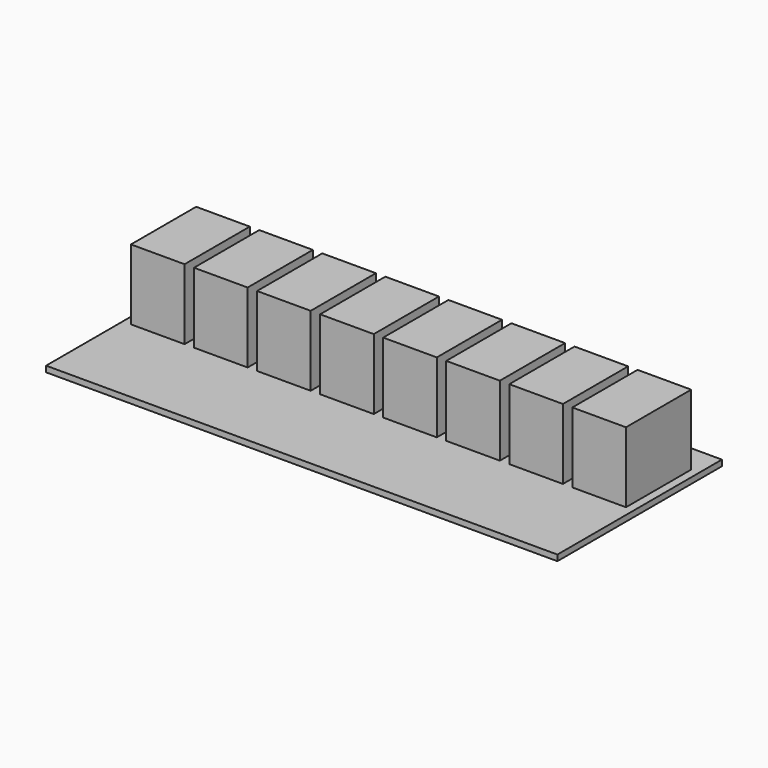
from build123d import *

# Parameters (mm, degrees)
F0_W     = 138
F0_H     = 55.5
F1_DEPTH = 1.5875
F2_W     = 14.4751365056
F2_H     = 21.9978075475
F3_DEPTH = 19


# Not quite as in the source:
# - a feature names something its author has since deleted; it is built from what else it names


with BuildPart() as f1:
    # F0 (on Top) → F1 (new body)
    with BuildSketch(Plane.XY):
        Rectangle(F0_W, F0_H)
    extrude(amount=F1_DEPTH)

    # F2 (on face) → F3 (join)
    with BuildSketch(Plane.XY.offset(1.5875)):
        with Locations((-25.527, 9.1310962263)):
            Rectangle(F2_W, F2_H)
        with Locations((-8.509, 9.1310962263)):
            Rectangle(F2_W, F2_H)
        with Locations((8.509, 9.1310962263)):
            Rectangle(F2_W, F2_H)
        with Locations((25.527, 9.1310962263)):
            Rectangle(F2_W, F2_H)
        with Locations((42.545, 9.1310962263)):
            Rectangle(F2_W, F2_H)
        with Locations((59.563, 9.1310962263)):
            Rectangle(F2_W, F2_H)
        with Locations((-42.545, 9.1310962263)):
            Rectangle(F2_W, F2_H)
        with Locations((-59.563, 9.1310962263)):
            Rectangle(F2_W, F2_H)
    extrude(amount=F3_DEPTH)


solid = f1.part
